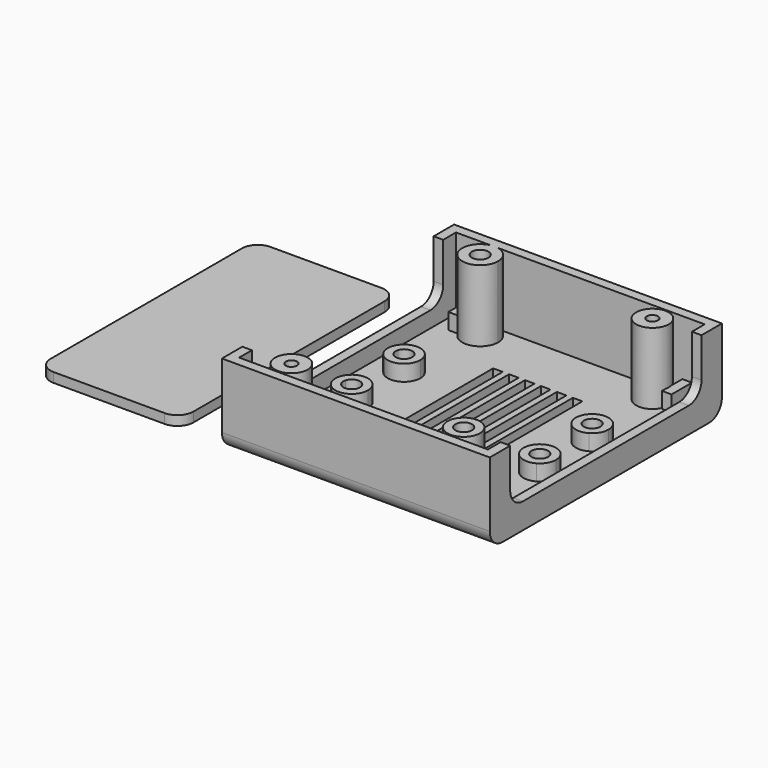
from build123d import *

# Parameters (mm, degrees)
F2_W      = 84
F2_H      = 91
F3_DEPTH  = 25.4
F4_T      = -3
F5_R      = 2.6
F5_R_2    = 5.1
F5_R_3    = 1.75
F6_DEPTH  = 22.4
F7_DEPTH  = 5
F9_DEPTH  = 5
F11_DEPTH = 5
F13_R     = 3
F14_DEPTH = 1.7
F15_R     = 5
F17_DEPTH = 3
F19_DEPTH = 3
F20_W     = 3
F20_H     = 51
F21_DEPTH = 3
F23_DEPTH = 3


with BuildPart() as f3:
    # F2 (on Top) → F3 (new body)
    with BuildSketch(Plane.XY):
        Rectangle(F2_W, F2_H)
    extrude(amount=F3_DEPTH)

    # F4
    f4_openings = [f3.faces().sort_by_distance(p)[0] for p in [
        (0, 0, 25.4),
    ]]
    offset(amount=F4_T, openings=f4_openings)

    # F5 (on face) → F6 (join, through all)
    with BuildSketch(Plane.XY.offset(3)):
        with BuildLine():
            ThreePointArc((-28.0625653753, 42.5), (-30.5769149302, 32.6837535924), (-21.409, 37))
            ThreePointArc((-21.409, 37), (-22.6927535924, 40.5679149302), (-25.9554346247, 42.5))
            Line((-25.9554346247, 42.5), (-28.0625653753, 42.5))
        make_face()
        with Locations((-27.009, 37)):
            Circle(F5_R, mode=Mode.SUBTRACT)
        with Locations((27.009, 37)):
            Circle(F5_R_2)
        with Locations((27.009, 37)):
            Circle(F5_R_3, mode=Mode.SUBTRACT)
        with Locations((-27.009, -37)):
            Circle(F5_R_2)
        with Locations((-27.009, -37)):
            Circle(F5_R_3, mode=Mode.SUBTRACT)
        with Locations((27.009, -37)):
            Circle(F5_R_2)
        with Locations((27.009, -37)):
            Circle(F5_R, mode=Mode.SUBTRACT)
    extrude(amount=F6_DEPTH)

    # F7 (cut): faces of the model
    f7_faces = [f3.faces().sort_by_distance(p)[0] for p in [
        (27.009, 37, 3),
        (-27.009, -37, 3),
    ]]
    extrude(f7_faces, amount=-F7_DEPTH, mode=Mode.SUBTRACT)

    # F8 (on face) → F9 (join)
    with BuildSketch(Plane.XY.offset(3)):
        with BuildLine():
            Line((-32, 42.5), (-35, 42.5))
            Line((-35, 42.5), (-35, 34.5))
            Line((-35, 34.5), (-32.0199879265, 34.5))
            ThreePointArc((-32.0199879265, 34.5), (-32.6089559562, 37.0222100909), (-32, 39.5396690729))
            Line((-32, 39.5396690729), (-32, 42.5))
        make_face()
        with BuildLine():
            Line((35, 42.5), (32, 42.5))
            Line((32, 42.5), (32, 38.0487702322))
            ThreePointArc((32, 38.0487702322), (32.0816768082, 37.5272096357), (32.109, 37))
            ThreePointArc((32.109, 37), (32.0816768082, 36.4727903643), (32, 35.9512297678))
            Line((32, 35.9512297678), (32, 34.5))
            Line((32, 34.5), (35, 34.5))
            Line((35, 34.5), (35, 42.5))
        make_face()
        with BuildLine():
            Line((32, -38.0487702322), (32, -42.5))
            Line((32, -42.5), (35, -42.5))
            Line((35, -42.5), (35, -34.5))
            Line((35, -34.5), (32, -34.5))
            Line((32, -34.5), (32, -35.9512297678))
            ThreePointArc((32, -35.9512297678), (32.0816768082, -36.4727903643), (32.109, -37))
            ThreePointArc((32.109, -37), (32.0816768082, -37.5272096357), (32, -38.0487702322))
        make_face()
        with BuildLine():
            Line((-35, -34.5), (-35, -42.5))
            Line((-35, -42.5), (-32, -42.5))
            Line((-32, -42.5), (-32, -38.0487702322))
            ThreePointArc((-32, -38.0487702322), (-32.109, -37), (-32, -35.9512297678))
            Line((-32, -35.9512297678), (-32, -34.5))
            Line((-32, -34.5), (-35, -34.5))
        make_face()
    extrude(amount=F9_DEPTH)

    # F10 (on face) → F11 (join)
    with BuildSketch(Plane.XY.offset(3)):
        with BuildLine():
            Line((-32, 10.9741428429), (-32, 14.7052221542))
            ThreePointArc((-32, 14.7052221542), (-34.6, 10.26), (-32, 5.8147778458))
            Line((-32, 5.8147778458), (-32, 9.5458571571))
            ThreePointArc((-32, 9.5458571571), (-32.1, 10.26), (-32, 10.9741428429))
        make_face()
        with BuildLine():
            ThreePointArc((-24.4, 10.26), (-26.9251213621, 14.6622721406), (-32, 14.7052221542))
            Line((-32, 14.7052221542), (-32, 10.9741428429))
            ThreePointArc((-32, 10.9741428429), (-29.1394448725, 12.8348786379), (-26.9, 10.26))
            ThreePointArc((-26.9, 10.26), (-29.1394448725, 7.6851213621), (-32, 9.5458571571))
            Line((-32, 9.5458571571), (-32, 5.8147778458))
            ThreePointArc((-32, 5.8147778458), (-26.9251213621, 5.8577278594), (-24.4, 10.26))
        make_face()
        with BuildLine():
            Line((32, 10.9741428429), (32, 14.7052221542))
            ThreePointArc((32, 14.7052221542), (24.4, 10.26), (32, 5.8147778458))
            Line((32, 5.8147778458), (32, 9.5458571571))
            ThreePointArc((32, 9.5458571571), (26.9, 10.26), (32, 10.9741428429))
        make_face()
        with BuildLine():
            ThreePointArc((34.6, 10.26), (33.9022721406, 12.8348786379), (32, 14.7052221542))
            Line((32, 14.7052221542), (32, 10.9741428429))
            ThreePointArc((32, 10.9741428429), (32.0748786379, 10.6205551275), (32.1, 10.26))
            ThreePointArc((32.1, 10.26), (32.0748786379, 9.8994448725), (32, 9.5458571571))
            Line((32, 9.5458571571), (32, 5.8147778458))
            ThreePointArc((32, 5.8147778458), (33.9022721406, 7.6851213621), (34.6, 10.26))
        make_face()
        with BuildLine():
            Line((32, -9.5458571571), (32, -5.8147778458))
            ThreePointArc((32, -5.8147778458), (24.4, -10.26), (32, -14.7052221542))
            Line((32, -14.7052221542), (32, -10.9741428429))
            ThreePointArc((32, -10.9741428429), (26.9, -10.26), (32, -9.5458571571))
        make_face()
        with BuildLine():
            ThreePointArc((34.6, -10.26), (33.9022721406, -7.6851213621), (32, -5.8147778458))
            Line((32, -5.8147778458), (32, -9.5458571571))
            ThreePointArc((32, -9.5458571571), (32.0748786379, -9.8994448725), (32.1, -10.26))
            ThreePointArc((32.1, -10.26), (32.0748786379, -10.6205551275), (32, -10.9741428429))
            Line((32, -10.9741428429), (32, -14.7052221542))
            ThreePointArc((32, -14.7052221542), (33.9022721406, -12.8348786379), (34.6, -10.26))
        make_face()
        with BuildLine():
            Line((-32, -9.5458571571), (-32, -5.8147778458))
            ThreePointArc((-32, -5.8147778458), (-34.6, -10.26), (-32, -14.7052221542))
            Line((-32, -14.7052221542), (-32, -10.9741428429))
            ThreePointArc((-32, -10.9741428429), (-32.1, -10.26), (-32, -9.5458571571))
        make_face()
        with BuildLine():
            ThreePointArc((-24.4, -10.26), (-26.9251213621, -5.8577278594), (-32, -5.8147778458))
            Line((-32, -5.8147778458), (-32, -9.5458571571))
            ThreePointArc((-32, -9.5458571571), (-29.1394448725, -7.6851213621), (-26.9, -10.26))
            ThreePointArc((-26.9, -10.26), (-29.1394448725, -12.8348786379), (-32, -10.9741428429))
            Line((-32, -10.9741428429), (-32, -14.7052221542))
            ThreePointArc((-32, -14.7052221542), (-26.9251213621, -14.6622721406), (-24.4, -10.26))
        make_face()
    extrude(amount=F11_DEPTH)

    # F13 (on face) → F14 (cut)
    with BuildSketch(Plane.XY):
        with Locations((-27, -37)):
            Circle(F13_R)
        with Locations((27, 37)):
            Circle(F13_R)
    extrude(amount=F14_DEPTH, mode=Mode.SUBTRACT)

    # F15
    f15_edges = [f3.edges().sort_by_distance(p)[0] for p in [
        (0, -45.5, 0),
        (0, 45.5, 0),
    ]]
    fillet(f15_edges, radius=F15_R)

    # F16 (on face) → F17 (cut)
    with BuildSketch(Plane(origin=(-42, 0, 0), x_dir=(0, -1, 0), z_dir=(-1, 0, 0))):
        with BuildLine():
            Line((-32.5, 8), (32.5, 8))
            ThreePointArc((32.5, 8), (36.0355339059, 9.4644660941), (37.5, 13))
            Line((37.5, 13), (37.5, 25.4))
            Line((37.5, 25.4), (-37.5, 25.4))
            Line((-37.5, 25.4), (-37.5, 13))
            ThreePointArc((-37.5, 13), (-36.0355339059, 9.4644660941), (-32.5, 8))
        make_face()
    extrude(amount=-F17_DEPTH, mode=Mode.SUBTRACT)

    # F18 (on face) → F19 (cut)
    with BuildSketch(Plane.YZ.offset(42)):
        with BuildLine():
            Line((37.5, 25.4), (-37.5, 25.4))
            Line((-37.5, 25.4), (-37.5, 13))
            ThreePointArc((-37.5, 13), (-36.0355339059, 9.4644660941), (-32.5, 8))
            Line((-32.5, 8), (32.5, 8))
            ThreePointArc((32.5, 8), (36.0355339059, 9.4644660941), (37.5, 13))
            Line((37.5, 13), (37.5, 25.4))
        make_face()
    extrude(amount=-F19_DEPTH, mode=Mode.SUBTRACT)

    # F20 (on face) → F21 (cut)
    with BuildSketch(Plane.XY):
        with Locations((-12.25, 0)):
            Rectangle(F20_W, F20_H)
        with Locations((-7.25, 0)):
            Rectangle(F20_W, F20_H)
        with Locations((-2.25, 0)):
            Rectangle(F20_W, F20_H)
        with Locations((2.75, 0)):
            Rectangle(F20_W, F20_H)
        with Locations((7.75, 0)):
            Rectangle(F20_W, F20_H)
        with Locations((12.75, 0)):
            Rectangle(F20_W, F20_H)
    extrude(amount=F21_DEPTH, mode=Mode.SUBTRACT)


with BuildPart() as f23:
    # F22 (on Top) → F23 (new body)
    with BuildSketch(Plane.XY):
        with BuildLine():
            ThreePointArc((-56.7323996544, 36.729978323), (-58.1968657485, 40.2655122289), (-61.7323996544, 41.729978323))
            Line((-61.7323996544, 41.729978323), (-96.5323996544, 41.729978323))
            ThreePointArc((-96.5323996544, 41.729978323), (-100.0679335603, 40.2655122289), (-101.5323996544, 36.729978323))
            Line((-101.5323996544, 36.729978323), (-101.5323996544, -38.270021677))
            ThreePointArc((-101.5323996544, -38.270021677), (-100.0679335603, -41.8055555829), (-96.5323996544, -43.270021677))
            Line((-96.5323996544, -43.270021677), (-61.7323996544, -43.270021677))
            ThreePointArc((-61.7323996544, -43.270021677), (-58.1968657485, -41.8055555829), (-56.7323996544, -38.270021677))
            Line((-56.7323996544, -38.270021677), (-56.7323996544, 36.729978323))
        make_face()
    extrude(amount=F23_DEPTH)


solid = Compound([f3.part, f23.part])
